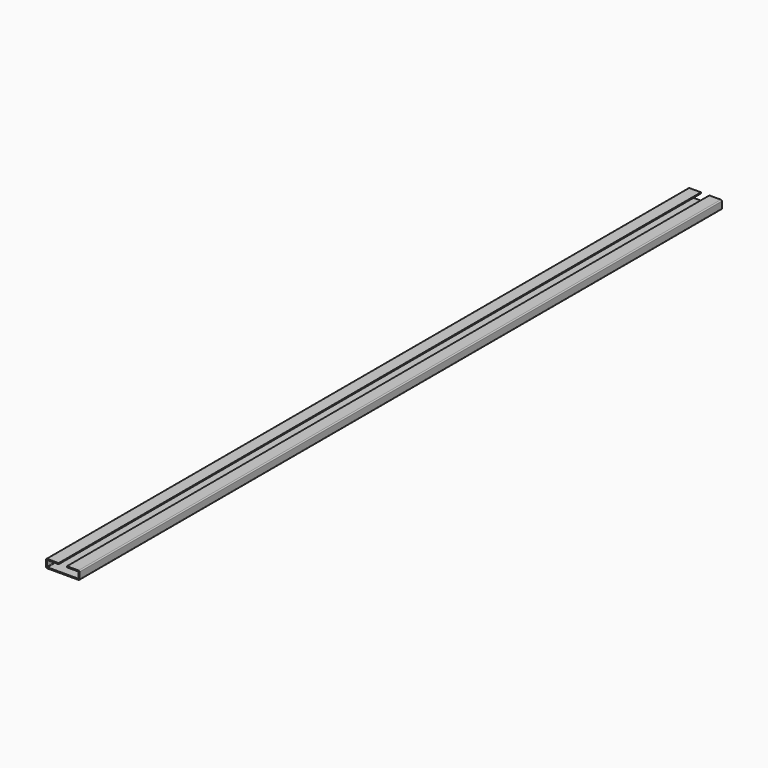
from build123d import *

# Parameters (mm, degrees)
F1_DEPTH = 1219.2
F2_R     = 0.79375
F3_R     = 1.5875


# Not quite as in the source:
# - a feature names something its author has since deleted; it is built from what else it names


with BuildPart() as f1:
    # F0 (on Front) → F1 (new body)
    with BuildSketch(Plane.XZ):
        Polygon((-25.4, 0), (0, 0), (25.4, 0), (25.4, 12.7), (6.35, 12.7), (6.35, 11.1125), (23.8125, 11.1125), (23.8125, 1.5875), (0, 1.5875), (-23.8125, 1.5875), (-23.8125, 11.1125), (-6.35, 11.1125), (-6.35, 12.7), (-25.4, 12.7), align=None)
    extrude(amount=F1_DEPTH)

    # F2
    f2_edges = [f1.edges().sort_by_distance(p)[0] for p in [
        (-23.8125, -609.6, 1.5875),
        (-23.8125, -609.6, 11.1125),
        (23.8125, -609.6, 1.5875),
        (23.8125, -609.6, 11.1125),
    ]]
    fillet(f2_edges, radius=F2_R)

    # F3
    f3_edges = [f1.edges().sort_by_distance(p)[0] for p in [
        (25.4, -609.6, 12.7),
        (25.4, -609.6, 0),
        (-25.4, -609.6, 0),
        (-25.4, -609.6, 12.7),
    ]]
    fillet(f3_edges, radius=F3_R)


solid = f1.part
